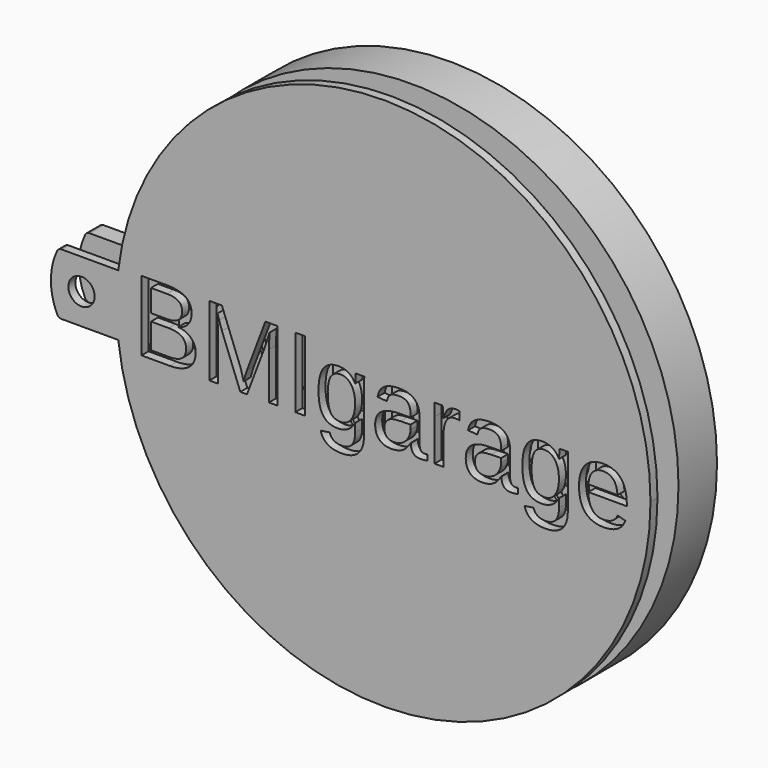
from build123d import *

# Parameters (mm, degrees)
F0_R          = 25.95
F0_R_2        = 24.75
F0_R_3        = 1.5
F1_DEPTH      = 2
F2_DEPTH      = 1
F3_DEPTH      = 3.5
F4_START      = -2.7
F4_DEPTH      = 0.8
F5_R          = 0.39999
F7_START      = 5
F7_DEPTH      = 1
F6_TEXT_SIZE  = 11.6359543791
F8_DEPTH      = 0.3
F8_DEPTH_BACK = 25
F9_T1_DEPTH   = 2
F9_T6_ANGLE   = 31.9656549812
F9_T13_DEPTH  = 6.3317787933
F9_T18_ANGLE  = 31.9656549812
F9_T25_DEPTH  = 6.3317787933
F9_T30_ANGLE  = 31.9656549812


# Not quite as in the source:
# - a fillet or chamfer that OpenCascade refuses, or shapes differently, is made with other operations: its cross-section is extruded or revolved along the edge and cut away or added
# - a fillet or chamfer is up to 0.001 mm smaller than in the source, because OpenCascade refuses the exact size
# - a feature names something its author has since deleted; it is built from what else it names
# - Text() gives the source's letters only with a copy of the font that has no kerning and outlines rounded to 1/6400 em; it was checked with that copy


with BuildPart() as f1:
    # F0 (on Front) → F1 (new body)
    with BuildSketch(Plane.XZ):
        with BuildLine():
            ThreePointArc((-30.2974528443, -3.5), (1.7528975374, -30.448530327), (30.4989450449, 0))
            ThreePointArc((30.4989450449, 0), (1.7528975374, 30.448530327), (-30.2974528443, 3.5))
            ThreePointArc((-30.2974528443, 3.5), (-30.4989450449, 0), (-30.2974528443, -3.5))
        make_face()
        with BuildLine():
            ThreePointArc((29.0669332201, 0.9977376368), (29.0797720736, 0.4989422432), (29.0840521113, 0))
            ThreePointArc((29.0840521113, 0), (29.0797720736, -0.4989422432), (29.0669332201, -0.9977376368))
            ThreePointArc((29.0669332201, -0.9977376368), (20.5655304723, -20.5655304723), (0.9977376368, -29.0669332201))
            ThreePointArc((0.9977376368, -29.0669332201), (0, -29.0840521113), (-0.9977376368, -29.0669332201))
            ThreePointArc((-0.9977376368, -29.0669332201), (-20.3380223428, -20.7905491605), (-29.0379433443, -1.6370502587))
            ThreePointArc((-29.0379433443, -1.6370502587), (-29.0840521113, 0), (-29.0379433443, 1.6370502587))
            ThreePointArc((-29.0379433443, 1.6370502587), (-20.3380223428, 20.7905491605), (-0.9977376368, 29.0669332201))
            ThreePointArc((-0.9977376368, 29.0669332201), (0, 29.0840521113), (0.9977376368, 29.0669332201))
            ThreePointArc((0.9977376368, 29.0669332201), (20.5655304723, 20.5655304723), (29.0669332201, 0.9977376368))
        make_face(mode=Mode.SUBTRACT)
        with BuildLine():
            Line((28.5107772126, 0.9977376368), (29.0669332201, 0.9977376368))
            ThreePointArc((29.0669332201, 0.9977376368), (20.5655304723, 20.5655304723), (0.9977376368, 29.0669332201))
            Line((0.9977376368, 29.0669332201), (0.9977376368, 28.5107772126))
            Line((0.9977376368, 28.5107772126), (-0.9977376368, 28.4669332201))
            Line((-0.9977376368, 28.4669332201), (-0.9977376368, 29.0669332201))
            ThreePointArc((-0.9977376368, 29.0669332201), (-20.3380223428, 20.7905491605), (-29.0379433443, 1.6370502587))
            Line((-29.0379433443, 1.6370502587), (-28.4817873368, 1.6370502587))
            Line((-28.4817873368, 1.6370502587), (-28.4817873368, -1.6370502587))
            Line((-28.4817873368, -1.6370502587), (-29.0379433443, -1.6370502587))
            ThreePointArc((-29.0379433443, -1.6370502587), (-20.3380223428, -20.7905491605), (-0.9977376368, -29.0669332201))
            Line((-0.9977376368, -29.0669332201), (-0.9977376368, -28.5107772126))
            Line((-0.9977376368, -28.5107772126), (0.9977376368, -28.5107772126))
            Line((0.9977376368, -28.5107772126), (0.9977376368, -29.0669332201))
            ThreePointArc((0.9977376368, -29.0669332201), (20.5655304723, -20.5655304723), (29.0669332201, -0.9977376368))
            Line((29.0669332201, -0.9977376368), (28.5107772126, -0.9977376368))
            Line((28.5107772126, -0.9977376368), (28.5107772126, 0.9977376368))
        make_face()
        Circle(F0_R, mode=Mode.SUBTRACT)
        Circle(F0_R)
        Circle(F0_R_2, mode=Mode.SUBTRACT)
        Circle(F0_R_2)
        with BuildLine():
            ThreePointArc((-30.2974528443, -3.5), (-30.4989450449, 0), (-30.2974528443, 3.5))
            Line((-30.2974528443, 3.5), (-36.7641973886, 3.5))
            ThreePointArc((-36.7641973886, 3.5), (-37.08347935, 3.4067688805), (-37.3024219268, 3.1563748697))
            ThreePointArc((-37.3024219268, 3.1563748697), (-37.9989450449, 0), (-37.3024219268, -3.1563748697))
            ThreePointArc((-37.3024219268, -3.1563748697), (-37.08347935, -3.4067688805), (-36.7641973886, -3.5))
            Line((-36.7641973886, -3.5), (-30.2974528443, -3.5))
        make_face()
        with Locations((-34.4989450449, 0)):
            Circle(F0_R_3, mode=Mode.SUBTRACT)
        with BuildLine():
            Line((-28.4817873368, 1.6370502587), (-29.0379433443, 1.6370502587))
            ThreePointArc((-29.0379433443, 1.6370502587), (-29.0840521113, 0), (-29.0379433443, -1.6370502587))
            Line((-29.0379433443, -1.6370502587), (-28.4817873368, -1.6370502587))
            Line((-28.4817873368, -1.6370502587), (-28.4817873368, 1.6370502587))
        make_face()
        with BuildLine():
            Line((0.9977376368, 28.5107772126), (0.9977376368, 29.0669332201))
            ThreePointArc((0.9977376368, 29.0669332201), (0, 29.0840521113), (-0.9977376368, 29.0669332201))
            Line((-0.9977376368, 29.0669332201), (-0.9977376368, 28.4669332201))
            Line((-0.9977376368, 28.4669332201), (0.9977376368, 28.5107772126))
        make_face()
        with BuildLine():
            ThreePointArc((-0.9977376368, -29.0669332201), (0, -29.0840521113), (0.9977376368, -29.0669332201))
            Line((0.9977376368, -29.0669332201), (0.9977376368, -28.5107772126))
            Line((0.9977376368, -28.5107772126), (-0.9977376368, -28.5107772126))
            Line((-0.9977376368, -28.5107772126), (-0.9977376368, -29.0669332201))
        make_face()
        with BuildLine():
            ThreePointArc((29.0669332201, -0.9977376368), (29.0797720736, -0.4989422432), (29.0840521113, 0))
            ThreePointArc((29.0840521113, 0), (29.0797720736, 0.4989422432), (29.0669332201, 0.9977376368))
            Line((29.0669332201, 0.9977376368), (28.5107772126, 0.9977376368))
            Line((28.5107772126, 0.9977376368), (28.5107772126, -0.9977376368))
            Line((28.5107772126, -0.9977376368), (29.0669332201, -0.9977376368))
        make_face()
    extrude(amount=F1_DEPTH)

    # F0 (on Front) → F2 (join)
    with BuildSketch(Plane.XZ):
        Circle(F0_R)
        Circle(F0_R_2, mode=Mode.SUBTRACT)
    extrude(amount=-F2_DEPTH)

    # F0 (on Front) → F3 (join)
    with BuildSketch(Plane.XZ):
        with BuildLine():
            ThreePointArc((-30.2974528443, -3.5), (1.7528975374, -30.448530327), (30.4989450449, 0))
            ThreePointArc((30.4989450449, 0), (1.7528975374, 30.448530327), (-30.2974528443, 3.5))
            ThreePointArc((-30.2974528443, 3.5), (-30.4989450449, 0), (-30.2974528443, -3.5))
        make_face()
        with BuildLine():
            ThreePointArc((29.0669332201, 0.9977376368), (29.0797720736, 0.4989422432), (29.0840521113, 0))
            ThreePointArc((29.0840521113, 0), (29.0797720736, -0.4989422432), (29.0669332201, -0.9977376368))
            ThreePointArc((29.0669332201, -0.9977376368), (20.5655304723, -20.5655304723), (0.9977376368, -29.0669332201))
            ThreePointArc((0.9977376368, -29.0669332201), (0, -29.0840521113), (-0.9977376368, -29.0669332201))
            ThreePointArc((-0.9977376368, -29.0669332201), (-20.3380223428, -20.7905491605), (-29.0379433443, -1.6370502587))
            ThreePointArc((-29.0379433443, -1.6370502587), (-29.0840521113, 0), (-29.0379433443, 1.6370502587))
            ThreePointArc((-29.0379433443, 1.6370502587), (-20.3380223428, 20.7905491605), (-0.9977376368, 29.0669332201))
            ThreePointArc((-0.9977376368, 29.0669332201), (0, 29.0840521113), (0.9977376368, 29.0669332201))
            ThreePointArc((0.9977376368, 29.0669332201), (20.5655304723, 20.5655304723), (29.0669332201, 0.9977376368))
        make_face(mode=Mode.SUBTRACT)
    extrude(amount=-F3_DEPTH)

    # F0 (on Front) → F4 (join)
    with BuildSketch(Plane.XZ.offset(F4_START)):
        with BuildLine():
            ThreePointArc((-0.9977376368, -29.0669332201), (0, -29.0840521113), (0.9977376368, -29.0669332201))
            Line((0.9977376368, -29.0669332201), (0.9977376368, -28.5107772126))
            Line((0.9977376368, -28.5107772126), (-0.9977376368, -28.5107772126))
            Line((-0.9977376368, -28.5107772126), (-0.9977376368, -29.0669332201))
        make_face()
        with BuildLine():
            ThreePointArc((29.0669332201, -0.9977376368), (29.0797720736, -0.4989422432), (29.0840521113, 0))
            ThreePointArc((29.0840521113, 0), (29.0797720736, 0.4989422432), (29.0669332201, 0.9977376368))
            Line((29.0669332201, 0.9977376368), (28.5107772126, 0.9977376368))
            Line((28.5107772126, 0.9977376368), (28.5107772126, -0.9977376368))
            Line((28.5107772126, -0.9977376368), (29.0669332201, -0.9977376368))
        make_face()
        with BuildLine():
            Line((-28.4817873368, 1.6370502587), (-29.0379433443, 1.6370502587))
            ThreePointArc((-29.0379433443, 1.6370502587), (-29.0840521113, 0), (-29.0379433443, -1.6370502587))
            Line((-29.0379433443, -1.6370502587), (-28.4817873368, -1.6370502587))
            Line((-28.4817873368, -1.6370502587), (-28.4817873368, 1.6370502587))
        make_face()
        with BuildLine():
            Line((0.9977376368, 28.5107772126), (0.9977376368, 29.0669332201))
            ThreePointArc((0.9977376368, 29.0669332201), (0, 29.0840521113), (-0.9977376368, 29.0669332201))
            Line((-0.9977376368, 29.0669332201), (-0.9977376368, 28.4669332201))
            Line((-0.9977376368, 28.4669332201), (0.9977376368, 28.5107772126))
        make_face()
    extrude(amount=-F4_DEPTH)

    # F5 (radius 0.4 in the source; OpenCascade refuses exactly that, so slightly less here)
    f5_edges = [f1.edges().sort_by_distance(p)[0] for p in [
        (0, 3.5, 28.488855),
        (0, 2.7, 28.488855),
        (-28.481787, 3.5, 0),
        (-28.481787, 2.7, 0),
        (0, 3.5, -28.510777),
        (0, 2.7, -28.510777),
        (28.510777, 3.5, 0),
        (28.510777, 2.7, 0),
    ]]
    fillet(f5_edges, radius=F5_R)


with BuildPart() as f7:
    # F0 (on Front) → F7 (new body)
    with BuildSketch(Plane.XZ.offset(F7_START)):
        with BuildLine():
            ThreePointArc((-30.2974528443, -3.5), (1.7528975374, -30.448530327), (30.4989450449, 0))
            ThreePointArc((30.4989450449, 0), (1.7528975374, 30.448530327), (-30.2974528443, 3.5))
            ThreePointArc((-30.2974528443, 3.5), (-30.4989450449, 0), (-30.2974528443, -3.5))
        make_face()
        with BuildLine():
            ThreePointArc((29.0669332201, 0.9977376368), (29.0797720736, 0.4989422432), (29.0840521113, 0))
            ThreePointArc((29.0840521113, 0), (29.0797720736, -0.4989422432), (29.0669332201, -0.9977376368))
            ThreePointArc((29.0669332201, -0.9977376368), (20.5655304723, -20.5655304723), (0.9977376368, -29.0669332201))
            ThreePointArc((0.9977376368, -29.0669332201), (0, -29.0840521113), (-0.9977376368, -29.0669332201))
            ThreePointArc((-0.9977376368, -29.0669332201), (-20.3380223428, -20.7905491605), (-29.0379433443, -1.6370502587))
            ThreePointArc((-29.0379433443, -1.6370502587), (-29.0840521113, 0), (-29.0379433443, 1.6370502587))
            ThreePointArc((-29.0379433443, 1.6370502587), (-20.3380223428, 20.7905491605), (-0.9977376368, 29.0669332201))
            ThreePointArc((-0.9977376368, 29.0669332201), (0, 29.0840521113), (0.9977376368, 29.0669332201))
            ThreePointArc((0.9977376368, 29.0669332201), (20.5655304723, 20.5655304723), (29.0669332201, 0.9977376368))
        make_face(mode=Mode.SUBTRACT)
        with BuildLine():
            Line((28.5107772126, 0.9977376368), (29.0669332201, 0.9977376368))
            ThreePointArc((29.0669332201, 0.9977376368), (20.5655304723, 20.5655304723), (0.9977376368, 29.0669332201))
            Line((0.9977376368, 29.0669332201), (0.9977376368, 28.5107772126))
            Line((0.9977376368, 28.5107772126), (-0.9977376368, 28.4669332201))
            Line((-0.9977376368, 28.4669332201), (-0.9977376368, 29.0669332201))
            ThreePointArc((-0.9977376368, 29.0669332201), (-20.3380223428, 20.7905491605), (-29.0379433443, 1.6370502587))
            Line((-29.0379433443, 1.6370502587), (-28.4817873368, 1.6370502587))
            Line((-28.4817873368, 1.6370502587), (-28.4817873368, -1.6370502587))
            Line((-28.4817873368, -1.6370502587), (-29.0379433443, -1.6370502587))
            ThreePointArc((-29.0379433443, -1.6370502587), (-20.3380223428, -20.7905491605), (-0.9977376368, -29.0669332201))
            Line((-0.9977376368, -29.0669332201), (-0.9977376368, -28.5107772126))
            Line((-0.9977376368, -28.5107772126), (0.9977376368, -28.5107772126))
            Line((0.9977376368, -28.5107772126), (0.9977376368, -29.0669332201))
            ThreePointArc((0.9977376368, -29.0669332201), (20.5655304723, -20.5655304723), (29.0669332201, -0.9977376368))
            Line((29.0669332201, -0.9977376368), (28.5107772126, -0.9977376368))
            Line((28.5107772126, -0.9977376368), (28.5107772126, 0.9977376368))
        make_face()
        Circle(F0_R, mode=Mode.SUBTRACT)
        Circle(F0_R)
        Circle(F0_R_2, mode=Mode.SUBTRACT)
        Circle(F0_R_2)
        with BuildLine():
            ThreePointArc((-30.2974528443, -3.5), (-30.4989450449, 0), (-30.2974528443, 3.5))
            Line((-30.2974528443, 3.5), (-36.7641973886, 3.5))
            ThreePointArc((-36.7641973886, 3.5), (-37.08347935, 3.4067688805), (-37.3024219268, 3.1563748697))
            ThreePointArc((-37.3024219268, 3.1563748697), (-37.9989450449, 0), (-37.3024219268, -3.1563748697))
            ThreePointArc((-37.3024219268, -3.1563748697), (-37.08347935, -3.4067688805), (-36.7641973886, -3.5))
            Line((-36.7641973886, -3.5), (-30.2974528443, -3.5))
        make_face()
        with Locations((-34.4989450449, 0)):
            Circle(F0_R_3, mode=Mode.SUBTRACT)
        with BuildLine():
            Line((-28.4817873368, 1.6370502587), (-29.0379433443, 1.6370502587))
            ThreePointArc((-29.0379433443, 1.6370502587), (-29.0840521113, 0), (-29.0379433443, -1.6370502587))
            Line((-29.0379433443, -1.6370502587), (-28.4817873368, -1.6370502587))
            Line((-28.4817873368, -1.6370502587), (-28.4817873368, 1.6370502587))
        make_face()
        with BuildLine():
            Line((0.9977376368, 28.5107772126), (0.9977376368, 29.0669332201))
            ThreePointArc((0.9977376368, 29.0669332201), (0, 29.0840521113), (-0.9977376368, 29.0669332201))
            Line((-0.9977376368, 29.0669332201), (-0.9977376368, 28.4669332201))
            Line((-0.9977376368, 28.4669332201), (0.9977376368, 28.5107772126))
        make_face()
        with BuildLine():
            ThreePointArc((29.0669332201, -0.9977376368), (29.0797720736, -0.4989422432), (29.0840521113, 0))
            ThreePointArc((29.0840521113, 0), (29.0797720736, 0.4989422432), (29.0669332201, 0.9977376368))
            Line((29.0669332201, 0.9977376368), (28.5107772126, 0.9977376368))
            Line((28.5107772126, 0.9977376368), (28.5107772126, -0.9977376368))
            Line((28.5107772126, -0.9977376368), (29.0669332201, -0.9977376368))
        make_face()
        with BuildLine():
            ThreePointArc((-0.9977376368, -29.0669332201), (0, -29.0840521113), (0.9977376368, -29.0669332201))
            Line((0.9977376368, -29.0669332201), (0.9977376368, -28.5107772126))
            Line((0.9977376368, -28.5107772126), (-0.9977376368, -28.5107772126))
            Line((-0.9977376368, -28.5107772126), (-0.9977376368, -29.0669332201))
        make_face()
    extrude(amount=F7_DEPTH)


with BuildPart() as f8_tool:
    # F6 (on face) → F8 (new body, two sides)
    with BuildSketch(Plane.XZ.offset(2)) as f8_sk:
        with Locations((-28.6026303582, -4.1889435765)):
            Text('BMIgarage', F6_TEXT_SIZE, font='Arimo', text_align=(TextAlign.LEFT, TextAlign.BOTTOM))
    extrude(amount=-F8_DEPTH)
    extrude(f8_sk.sketch, amount=F8_DEPTH_BACK)


with BuildPart() as f1_1:
    add(f1.part)

    # F8: cut by f8_tool
    add(f8_tool.part, mode=Mode.SUBTRACT)

    # F9: fillet of radius 2 on 3 edges, made by hand

    # F9_s2 → F9_t1 (join)
    with BuildSketch(Plane.XZ):
        with BuildLine():
            ThreePointArc((-30.0590133401, 5.1615274747), (-30.7411618501, 3.9707934981), (-32.0301643616, 3.5))
            Line((-32.0301643616, 3.5), (-30.2974528443, 3.5))
            ThreePointArc((-30.2974528443, 3.5), (-30.1896657974, 4.3324044015), (-30.0590133401, 5.1615274747))
        make_face()
        with BuildLine():
            ThreePointArc((-30.0590133401, -5.1615274747), (-30.7411618501, -3.9707934981), (-32.0301643616, -3.5))
            Line((-32.0301643616, -3.5), (-30.2974528443, -3.5))
            ThreePointArc((-30.2974528443, -3.5), (-30.1896657974, -4.3324044015), (-30.0590133401, -5.1615274747))
        make_face()
    extrude(amount=F9_T1_DEPTH)


with BuildPart() as f7_1:
    add(f7.part)

    # F8: cut by f8_tool
    add(f8_tool.part, mode=Mode.SUBTRACT)


with BuildPart() as f9_tool4:
    # F9_s5 → F9_t6 (revolve)
    with BuildSketch(Plane(origin=(0, 0, 0), x_dir=(0, 1, 0), z_dir=(0.2753492371, 0, -0.9613442659))):
        with BuildLine():
            ThreePointArc((2, -30.4989450449), (0.5857864376, -31.0847314826), (0, -32.4989450449))
            Line((0, -32.4989450449), (0, -30.4989450449))
            Line((0, -30.4989450449), (2, -30.4989450449))
        make_face()
    revolve(axis=Axis((0, 0, 0), (0, 1, 0)), revolution_arc=F9_T6_ANGLE)

    split(bisect_by=Plane.XY.offset(-3.5), keep=Keep.TOP)

    split(bisect_by=Plane.XY.offset(3.5), keep=Keep.BOTTOM)


with BuildPart() as f1_2:
    add(f1_1.part)

    # F9_t3: union F9_tool4
    add(f9_tool4.part)


with BuildPart() as f9_tool11:
    # F9_s12 → F9_t13 (new body)
    with BuildSketch(Plane.XZ.offset(-4.3317787933)):
        with BuildLine():
            ThreePointArc((-30.0590133401, -5.1615274747), (-30.7411618501, -3.9707934981), (-32.0301643616, -3.5))
            Line((-32.0301643616, -3.5), (-30.2974528443, -3.5))
            ThreePointArc((-30.2974528443, -3.5), (-30.1896657974, -4.3324044015), (-30.0590133401, -5.1615274747))
        make_face()
    extrude(amount=F9_T13_DEPTH)

    split(bisect_by=Plane.XZ.offset(-3.5), keep=Keep.TOP)

    split(bisect_by=Plane.XZ, keep=Keep.BOTTOM)


with BuildPart() as f9_tool16:
    # F9_s17 → F9_t18 (revolve)
    with BuildSketch(Plane(origin=(0, 0, 0), x_dir=(0, 1, 0), z_dir=(0.2753492371, 0, -0.9613442659))):
        with BuildLine():
            ThreePointArc((2, -30.4989450449), (0.5857864376, -31.0847314826), (0, -32.4989450449))
            Line((0, -32.4989450449), (0, -30.4989450449))
            Line((0, -30.4989450449), (2, -30.4989450449))
        make_face()
    revolve(axis=Axis((0, 0, 0), (0, 1, 0)), revolution_arc=F9_T18_ANGLE)

    split(bisect_by=Plane.XY.offset(-3.5), keep=Keep.BOTTOM)


with BuildPart() as f9_tool11_1:
    add(f9_tool11.part)

    # F9_t20: intersect F9_tool16
    add(f9_tool16.part, mode=Mode.INTERSECT)


with BuildPart() as f1_3:
    add(f1_2.part)

    # F9_t9: union F9_tool11
    add(f9_tool11_1.part)


with BuildPart() as f9_tool23:
    # F9_s24 → F9_t25 (new body)
    with BuildSketch(Plane.XZ.offset(-4.3317787933)):
        with BuildLine():
            ThreePointArc((-30.0590133401, 5.1615274747), (-30.7411618501, 3.9707934981), (-32.0301643616, 3.5))
            Line((-32.0301643616, 3.5), (-30.2974528443, 3.5))
            ThreePointArc((-30.2974528443, 3.5), (-30.1896657974, 4.3324044015), (-30.0590133401, 5.1615274747))
        make_face()
    extrude(amount=F9_T25_DEPTH)

    split(bisect_by=Plane.XZ.offset(-3.5), keep=Keep.TOP)

    split(bisect_by=Plane.XZ, keep=Keep.BOTTOM)


with BuildPart() as f9_tool28:
    # F9_s29 → F9_t30 (revolve)
    with BuildSketch(Plane(origin=(0, 0, 0), x_dir=(0, 1, 0), z_dir=(0.2753492371, 0, -0.9613442659))):
        with BuildLine():
            ThreePointArc((2, -30.4989450449), (0.5857864376, -31.0847314826), (0, -32.4989450449))
            Line((0, -32.4989450449), (0, -30.4989450449))
            Line((0, -30.4989450449), (2, -30.4989450449))
        make_face()
    revolve(axis=Axis((0, 0, 0), (0, 1, 0)), revolution_arc=F9_T30_ANGLE)

    split(bisect_by=Plane.XY.offset(3.5), keep=Keep.TOP)


with BuildPart() as f9_tool23_1:
    add(f9_tool23.part)

    # F9_t32: intersect F9_tool28
    add(f9_tool28.part, mode=Mode.INTERSECT)


with BuildPart() as f1_4:
    add(f1_3.part)

    # F9_t21: union F9_tool23
    add(f9_tool23_1.part)


solid = Compound([f7_1.part, f1_4.part])
